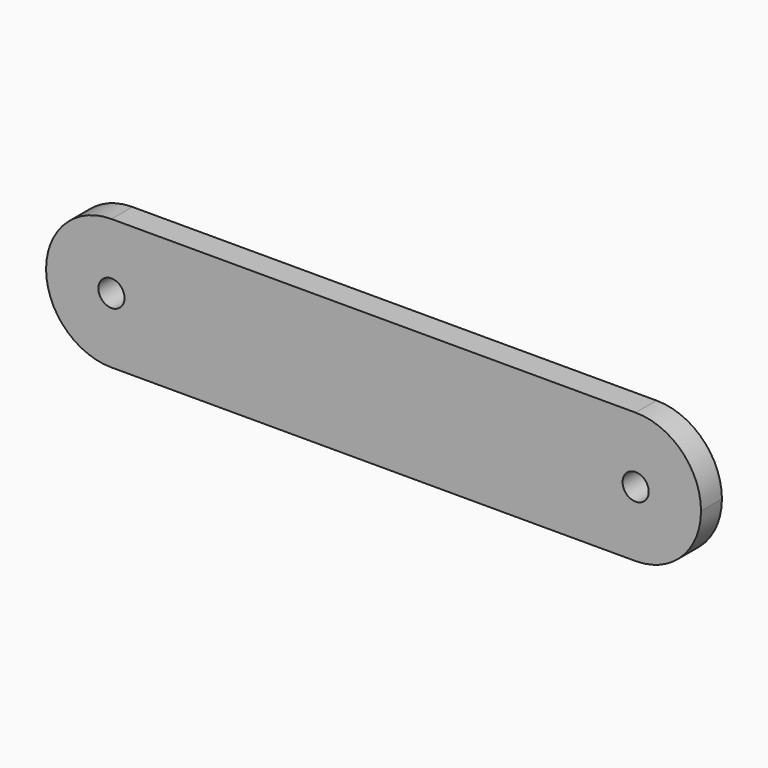
from build123d import *

# Parameters (mm, degrees)
F0_W     = 50.1
F0_H     = 10
F0_R     = 1
F1_DEPTH = 2
F2_R     = 4.99999


# Not quite as in the source:
# - a fillet or chamfer is up to 0.001 mm smaller than in the source, because OpenCascade refuses the exact size


with BuildPart() as f1:
    # F0 (on Front) → F1 (new body)
    with BuildSketch(Plane.XZ):
        with Locations((25.05, -5)):
            Rectangle(F0_W, F0_H)
        with Locations((5, -5)):
            Circle(F0_R, mode=Mode.SUBTRACT)
        with Locations((45.1, -5)):
            Circle(F0_R, mode=Mode.SUBTRACT)
    extrude(amount=F1_DEPTH)

    # F2 (radius 5 in the source; OpenCascade refuses exactly that, so slightly less here)
    f2_edges = [f1.edges().sort_by_distance(p)[0] for p in [
        (0, -1, 0),
        (0, -1, -10),
        (50.1, -1, 0),
        (50.1, -1, -10),
    ]]
    fillet(f2_edges, radius=F2_R)


solid = f1.part
